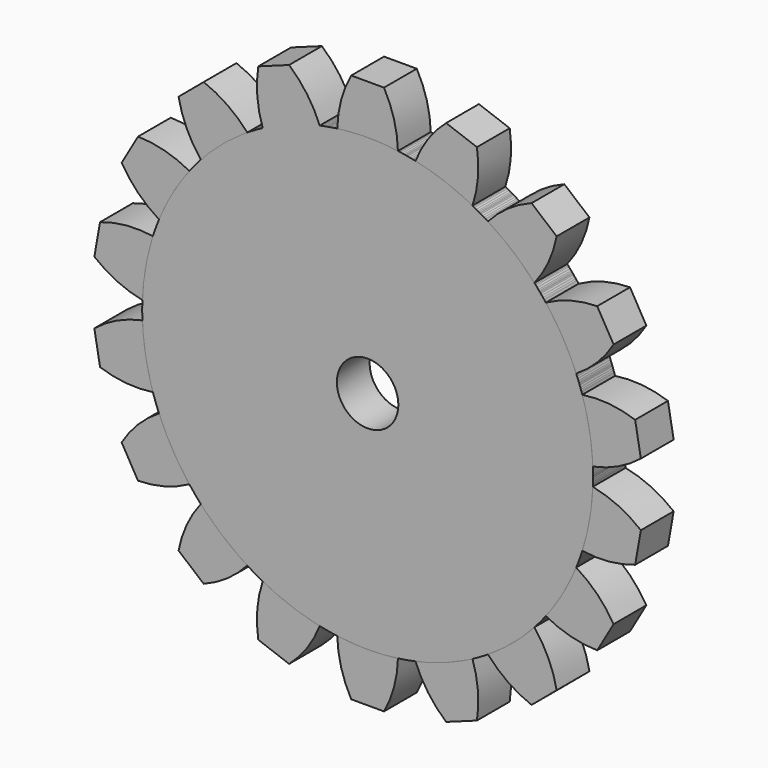
from build123d import *

# Parameters (mm, degrees)
F1_DEPTH = 6.35
F2_COUNT = 18
F3_R     = 9.525
F4_DEPTH = 12.701


# Not quite as in the source:
# - a feature names something its author has since deleted; it is built from what else it names


with BuildPart() as f1:
    # F0 (on Front) → F1 (new body, symmetric)
    with BuildSketch(Plane.XZ):
        with BuildLine():
            ThreePointArc((-9.3971418527, 69.215), (-45.9490595202, -52.6089957061), (69.85, 0))
            ThreePointArc((69.85, 0), (52.6089957061, 45.9490595202), (9.3971418527, 69.215))
            ThreePointArc((9.3971418527, 69.215), (4.7092860393, 69.6910691911), (0, 69.85))
            ThreePointArc((0, 69.85), (-4.7092860393, 69.6910691911), (-9.3971418527, 69.215))
        make_face()
        with BuildLine():
            ThreePointArc((0, 69.85), (4.7092860393, 69.6910691911), (9.3971418527, 69.215))
            ThreePointArc((9.3971418527, 69.215), (8.2047336853, 77.415244043), (5.08, 85.09))
            Line((5.08, 85.09), (-5.08, 85.09))
            ThreePointArc((-5.08, 85.09), (-8.2047336853, 77.415244043), (-9.3971418527, 69.215))
            ThreePointArc((-9.3971418527, 69.215), (-4.7092860393, 69.6910691911), (0, 69.85))
        make_face()
    extrude(amount=F1_DEPTH, both=True)


with BuildPart() as f2_1:
    # F2: instance of F1
    add(f1.part.rotate(Axis((0, 0, 0), (0, 1, 0)), 1 * 360 / F2_COUNT))


with BuildPart() as f2_2:
    # F2: instance of F1
    add(f1.part.rotate(Axis((0, 0, 0), (0, 1, 0)), 2 * 360 / F2_COUNT))


with BuildPart() as f2_3:
    # F2: instance of F1
    add(f1.part.rotate(Axis((0, 0, 0), (0, 1, 0)), 3 * 360 / F2_COUNT))


with BuildPart() as f2_4:
    # F2: instance of F1
    add(f1.part.rotate(Axis((0, 0, 0), (0, 1, 0)), 4 * 360 / F2_COUNT))


with BuildPart() as f2_5:
    # F2: instance of F1
    add(f1.part.rotate(Axis((0, 0, 0), (0, 1, 0)), 5 * 360 / F2_COUNT))


with BuildPart() as f2_6:
    # F2: instance of F1
    add(f1.part.rotate(Axis((0, 0, 0), (0, 1, 0)), 6 * 360 / F2_COUNT))


with BuildPart() as f2_7:
    # F2: instance of F1
    add(f1.part.rotate(Axis((0, 0, 0), (0, 1, 0)), 7 * 360 / F2_COUNT))


with BuildPart() as f2_8:
    # F2: instance of F1
    add(f1.part.rotate(Axis((0, 0, 0), (0, 1, 0)), 8 * 360 / F2_COUNT))


with BuildPart() as f2_9:
    # F2: instance of F1
    add(f1.part.rotate(Axis((0, 0, 0), (0, 1, 0)), 9 * 360 / F2_COUNT))


with BuildPart() as f2_10:
    # F2: instance of F1
    add(f1.part.rotate(Axis((0, 0, 0), (0, 1, 0)), 10 * 360 / F2_COUNT))


with BuildPart() as f2_11:
    # F2: instance of F1
    add(f1.part.rotate(Axis((0, 0, 0), (0, 1, 0)), 11 * 360 / F2_COUNT))


with BuildPart() as f2_12:
    # F2: instance of F1
    add(f1.part.rotate(Axis((0, 0, 0), (0, 1, 0)), 12 * 360 / F2_COUNT))


with BuildPart() as f2_13:
    # F2: instance of F1
    add(f1.part.rotate(Axis((0, 0, 0), (0, 1, 0)), 13 * 360 / F2_COUNT))


with BuildPart() as f2_14:
    # F2: instance of F1
    add(f1.part.rotate(Axis((0, 0, 0), (0, 1, 0)), 14 * 360 / F2_COUNT))


with BuildPart() as f2_15:
    # F2: instance of F1
    add(f1.part.rotate(Axis((0, 0, 0), (0, 1, 0)), 15 * 360 / F2_COUNT))


with BuildPart() as f2_16:
    # F2: instance of F1
    add(f1.part.rotate(Axis((0, 0, 0), (0, 1, 0)), 16 * 360 / F2_COUNT))


with BuildPart() as f2_17:
    # F2: instance of F1
    add(f1.part.rotate(Axis((0, 0, 0), (0, 1, 0)), 17 * 360 / F2_COUNT))


with BuildPart() as f4_tool:
    # F3 (on face) → F4 (new body, through all)
    with BuildSketch(Plane.XZ.offset(6.35)):
        Circle(F3_R)
    extrude(amount=-F4_DEPTH)


with BuildPart() as f1_1:
    add(f1.part)

    # F4: cut by f4_tool
    add(f4_tool.part, mode=Mode.SUBTRACT)


with BuildPart() as f2_1_1:
    add(f2_1.part)

    # F4: cut by f4_tool
    add(f4_tool.part, mode=Mode.SUBTRACT)


with BuildPart() as f2_2_1:
    add(f2_2.part)

    # F4: cut by f4_tool
    add(f4_tool.part, mode=Mode.SUBTRACT)


with BuildPart() as f2_3_1:
    add(f2_3.part)

    # F4: cut by f4_tool
    add(f4_tool.part, mode=Mode.SUBTRACT)


with BuildPart() as f2_4_1:
    add(f2_4.part)

    # F4: cut by f4_tool
    add(f4_tool.part, mode=Mode.SUBTRACT)


with BuildPart() as f2_5_1:
    add(f2_5.part)

    # F4: cut by f4_tool
    add(f4_tool.part, mode=Mode.SUBTRACT)


with BuildPart() as f2_6_1:
    add(f2_6.part)

    # F4: cut by f4_tool
    add(f4_tool.part, mode=Mode.SUBTRACT)


with BuildPart() as f2_7_1:
    add(f2_7.part)

    # F4: cut by f4_tool
    add(f4_tool.part, mode=Mode.SUBTRACT)


with BuildPart() as f2_8_1:
    add(f2_8.part)

    # F4: cut by f4_tool
    add(f4_tool.part, mode=Mode.SUBTRACT)


with BuildPart() as f2_9_1:
    add(f2_9.part)

    # F4: cut by f4_tool
    add(f4_tool.part, mode=Mode.SUBTRACT)


with BuildPart() as f2_10_1:
    add(f2_10.part)

    # F4: cut by f4_tool
    add(f4_tool.part, mode=Mode.SUBTRACT)


with BuildPart() as f2_11_1:
    add(f2_11.part)

    # F4: cut by f4_tool
    add(f4_tool.part, mode=Mode.SUBTRACT)


with BuildPart() as f2_12_1:
    add(f2_12.part)

    # F4: cut by f4_tool
    add(f4_tool.part, mode=Mode.SUBTRACT)


with BuildPart() as f2_13_1:
    add(f2_13.part)

    # F4: cut by f4_tool
    add(f4_tool.part, mode=Mode.SUBTRACT)


with BuildPart() as f2_14_1:
    add(f2_14.part)

    # F4: cut by f4_tool
    add(f4_tool.part, mode=Mode.SUBTRACT)


with BuildPart() as f2_15_1:
    add(f2_15.part)

    # F4: cut by f4_tool
    add(f4_tool.part, mode=Mode.SUBTRACT)


with BuildPart() as f2_16_1:
    add(f2_16.part)

    # F4: cut by f4_tool
    add(f4_tool.part, mode=Mode.SUBTRACT)


with BuildPart() as f2_17_1:
    add(f2_17.part)

    # F4: cut by f4_tool
    add(f4_tool.part, mode=Mode.SUBTRACT)


solid = Compound([f1_1.part, f2_1_1.part, f2_2_1.part, f2_3_1.part, f2_4_1.part, f2_5_1.part, f2_6_1.part, f2_7_1.part, f2_8_1.part, f2_9_1.part, f2_10_1.part, f2_11_1.part, f2_12_1.part, f2_13_1.part, f2_14_1.part, f2_15_1.part, f2_16_1.part, f2_17_1.part])
